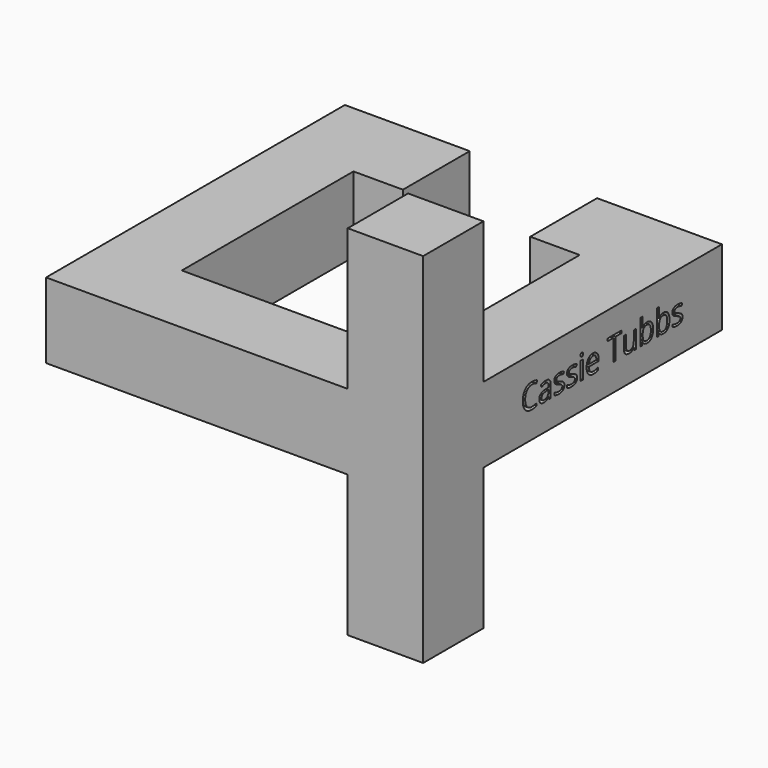
from build123d import *

# Parameters (mm, degrees)
F0_W         = 40
F0_H         = 40
F1_DEPTH     = 40
F5_DEPTH     = 40
F6_DEPTH     = 40
F4_W         = 32
F4_H         = 16
F7_DEPTH     = 40
F8_TEXT_SIZE = 3.5420209903
F9_DEPTH     = 5
F10_DEPTH    = 40


# Not quite as in the source:
# - a feature names something its author has since deleted; it is built from what else it names
# - Text() gives the source's letters only with a copy of the font that has no kerning and outlines rounded to 1/6400 em; it was checked with that copy


with BuildPart() as f1:
    # F0 (on Top) → F1 (new body)
    with BuildSketch(Plane.XY):
        Rectangle(F0_W, F0_H)
    extrude(amount=-F1_DEPTH)

    # F2 (on face) → F5 (cut)
    with BuildSketch(Plane.XY):
        Polygon((-20, 20), (-20, 19.6190571785), (-6.7529523894, 19.6190571785), (-6.7529523894, 10.7595995069), (-12, 10.7595995069), (-12, -12), (12, -12), (12, 10.7595995069), (6.7529523894, 10.7595995069), (6.7529523894, 19.6190571785), (20, 19.6190571785), (20, 20), align=None)
    extrude(amount=-F5_DEPTH, mode=Mode.SUBTRACT)

    # F3 (on face) → F6 (cut)
    with BuildSketch(Plane.XZ.offset(20)):
        Polygon((-20, 0), (-20, -16), (12, -16), (12, -1), (20, -1), (20, 0), align=None)
    extrude(amount=-F6_DEPTH, mode=Mode.SUBTRACT)

    # F4 (on face) → F7 (cut)
    with BuildSketch(Plane.YZ.offset(20)):
        with Locations((4, -8)):
            Rectangle(F4_W, F4_H)
        with Locations((4, -32)):
            Rectangle(F4_W, F4_H)
    extrude(amount=-F7_DEPTH, mode=Mode.SUBTRACT)

    # F8 (on face) → F9 (cut)
    with BuildSketch(Plane.YZ.offset(20)):
        with Locations((-7, -21.1584549988)):
            Text('Cassie Tubbs', F8_TEXT_SIZE, font='Open Sans', text_align=(TextAlign.LEFT, TextAlign.BOTTOM))
    extrude(amount=-F9_DEPTH, mode=Mode.SUBTRACT)

    # F3 (on face) → F10 (cut)
    with BuildSketch(Plane.XZ.offset(20)):
        Polygon((12, -39), (12, -24), (-20, -24), (-20, -40), (20, -40), (20, -39), align=None)
    extrude(amount=-F10_DEPTH, mode=Mode.SUBTRACT)


solid = f1.part
